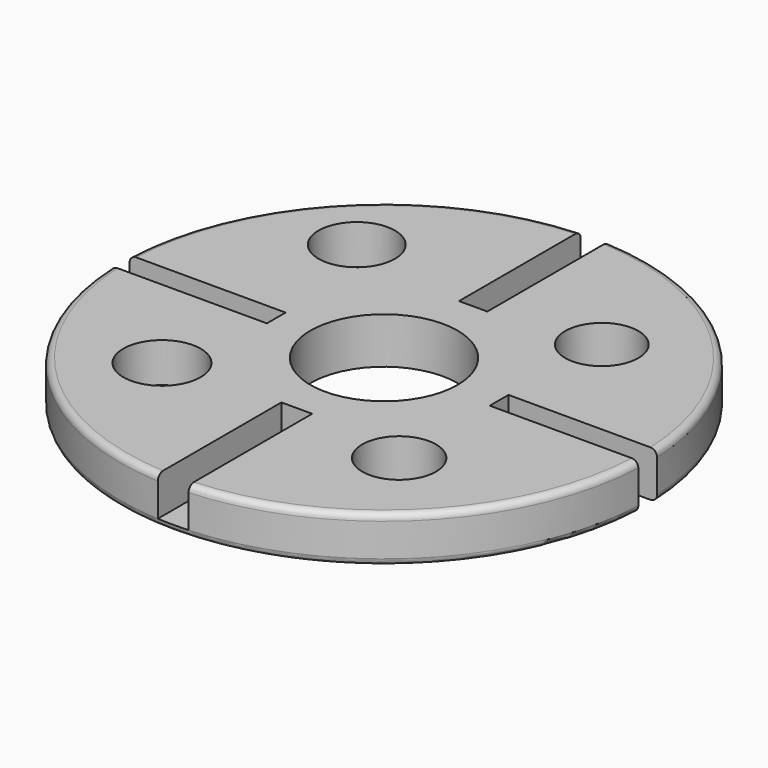
from build123d import *

# Parameters (mm, degrees)
F0_R      = 40
F0_R_2    = 11.15
F1_DEPTH  = 7
F3_W      = 4.2920620181
F3_H      = 25.3791473806
F4_DEPTH  = 50
F5_W      = 38.4419448674
F5_H      = 3.5456162877
F6_DEPTH  = 25
F8_W      = 29.4845998287
F8_H      = 3.5456162877
F9_DEPTH  = 25
F12_R     = 1
F13_DEPTH = 6
F10_R     = 5.7969793016
F10_R_2   = 5.8597151437
F11_R     = 5.5483568343
F11_R_2   = 5.5921159978
F14_DEPTH = 6


with BuildPart() as f1:
    # F0 (on Top) → F1 (new body)
    with BuildSketch(Plane.XY):
        Circle(F0_R)
        Circle(F0_R_2, mode=Mode.SUBTRACT)
    extrude(amount=F1_DEPTH)

    # F3 (on face) → F4 (cut)
    with BuildSketch(Plane.XY.offset(7)):
        with Locations((0, 29.5779034495)):
            Rectangle(F3_W, F3_H)
    extrude(amount=-F4_DEPTH, mode=Mode.SUBTRACT)

    # F5 (on face) → F6 (cut)
    with BuildSketch(Plane.XY.offset(7)):
        with Locations((-35.5494692922, 0)):
            Rectangle(F5_W, F5_H)
    extrude(amount=-F6_DEPTH, mode=Mode.SUBTRACT)

    # F8 (on face) → F9 (cut)
    with BuildSketch(Plane.XY.offset(7)):
        with Locations((32.1904607117, 0)):
            Rectangle(F8_W, F8_H)
    extrude(amount=-F9_DEPTH, mode=Mode.SUBTRACT)

    # F12
    f12_edges = [f1.edges().sort_by_distance(p)[0] for p in [
        (-28.416076, 28.15185, 7),
        (-28.416076, 28.15185, 0),
        (0, -40, 0),
        (28.416076, 28.15185, 0),
        (0, -40, 7),
        (28.416076, 28.15185, 7),
    ]]
    fillet(f12_edges, radius=F12_R)

    # F7 (on face) → F13 (cut)
    with BuildSketch(Plane.XY.offset(7)):
        with BuildLine():
            ThreePointArc((-2.3326422088, -39.9319268296), (0, -40), (2.3326422088, -39.9319268296))
            Line((2.3326422088, -39.9319268296), (2.3326422088, -16.5151059628))
            Line((2.3326422088, -16.5151059628), (-2.3326422088, -16.5151059628))
            Line((-2.3326422088, -16.5151059628), (-2.3326422088, -39.9319268296))
        make_face()
    extrude(amount=-F13_DEPTH, mode=Mode.SUBTRACT)

    # F10 (on face) + F11 (on face) → F14 (cut)
    with BuildSketch(Plane.XY.offset(7)):
        with Locations((-20.6205584109, 20.6205565482)):
            Circle(F10_R)
        with Locations((-19.687499851, -17.4481645226)):
            Circle(F10_R_2)
    with BuildSketch(Plane.XY.offset(7)):
        with Locations((18.0079955608, 18.7544431537)):
            Circle(F11_R)
        with Locations((17.4481645226, -18.9410559833)):
            Circle(F11_R_2)
    extrude(amount=-F14_DEPTH, mode=Mode.SUBTRACT)


solid = f1.part
